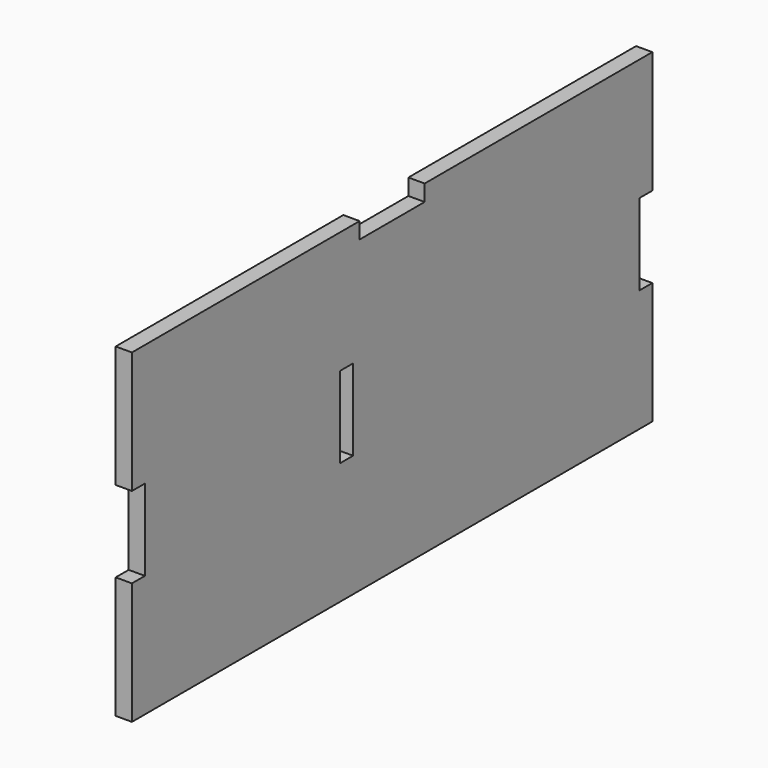
from build123d import *

# Parameters (mm, degrees)
F0_W     = 5
F0_H     = 25
F1_DEPTH = 5


# Not quite as in the source:
# - a feature names something its author has since deleted; it is built from what else it names


with BuildPart() as f1:
    # F0 (on Right) → F1 (new body)
    with BuildSketch(Plane.YZ):
        Polygon((138.9010111106, 39.8091464203), (138.9010111106, 77.3091464203), (51.4010111106, 77.3091464203), (51.4010111106, 72.3091464203), (26.4010111106, 72.3091464203), (26.4010111106, 77.3091464203), (-61.0989888894, 77.3091464203), (-61.0989888894, 39.8091464203), (-56.0989888894, 39.8091464203), (-56.0989888894, 14.8091464203), (-61.0989888894, 14.8091464203), (-61.0989888894, -22.6908535797), (138.9010111106, -22.6908535797), (138.9010111106, 14.8091464203), (133.9010111106, 14.8091464203), (133.9010111106, 39.8091464203), align=None)
        with Locations((21.4010111106, 27.3091464203)):
            Rectangle(F0_W, F0_H, mode=Mode.SUBTRACT)
    extrude(amount=F1_DEPTH)


solid = f1.part
